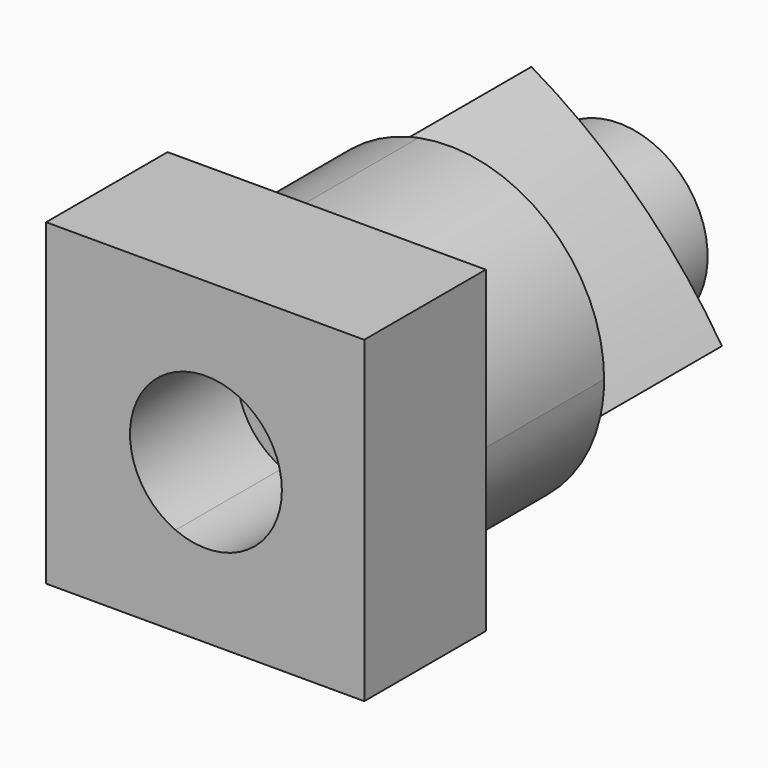
from build123d import *
from build123d import SkipClean  # not in build123d's __all__

# Parameters (mm, degrees)
F1_DEPTH = 6.35
F2_W     = 13.3050326258
F2_H     = 13.3050344884
F2_R     = 6.4893385046
F3_DEPTH = 6.35
F4_DEPTH = 25.4
F5_DEPTH = 7.112
F7_DEPTH = 6.35
F8_R     = 3.7056239581
F9_DEPTH = 2.54


# Not quite as in the source:
# - after a boolean that leaves OpenCascade's solid faulty, fix() repairs it


with BuildPart() as f1:
    # F0 (on Front) → F1 (new body)
    with BuildSketch(Plane.XZ):
        with BuildLine():
            ThreePointArc((-31.8034514785, 8.237525334), (-33.7084514785, 11.1474609002), (-31.8034514785, 14.0573964665))
            Line((-31.8034514785, 14.0573964665), (-31.8034514785, 17.5113130534))
            ThreePointArc((-31.8034514785, 17.5113130534), (-37.0227899831, 11.1474609002), (-31.8034514785, 4.7836087471))
            Line((-31.8034514785, 4.7836087471), (-31.8034514785, 8.237525334))
        make_face()
        with BuildLine():
            Line((-31.8034514785, 8.237525334), (-31.8034514785, 14.0573964665))
            ThreePointArc((-31.8034514785, 14.0573964665), (-33.7084514785, 11.1474609002), (-31.8034514785, 8.237525334))
        make_face()
        with BuildLine():
            ThreePointArc((-31.8034514785, 14.0573964665), (-28.7944323584, 13.8038564845), (-27.3584514785, 11.1474609002))
            ThreePointArc((-27.3584514785, 11.1474609002), (-28.7944323584, 8.491065316), (-31.8034514785, 8.237525334))
            Line((-31.8034514785, 8.237525334), (-31.8034514785, 4.7836087471))
            ThreePointArc((-31.8034514785, 4.7836087471), (-26.4182325094, 6.129843232), (-24.0441129739, 11.1474609002))
            ThreePointArc((-24.0441129739, 11.1474609002), (-26.4182325094, 16.1650785684), (-31.8034514785, 17.5113130534))
            Line((-31.8034514785, 17.5113130534), (-31.8034514785, 14.0573964665))
        make_face()
    extrude(amount=F1_DEPTH)

    # F2 (on face) → F3 (join)
    with BuildSketch(Plane.XZ.offset(6.35)):
        with Locations((-30.5656185374, 11.1557710916)):
            Rectangle(F2_W, F2_H)
        with Locations((-30.5334514785, 11.1474609002)):
            Circle(F2_R, mode=Mode.SUBTRACT)
        with Locations((-30.5334514785, 11.1474609002)):
            Circle(F2_R)
        with BuildLine():
            ThreePointArc((-31.8034514785, 14.0573964665), (-27.3584514785, 11.1474609002), (-31.8034514785, 8.237525334))
            Line((-31.8034514785, 8.237525334), (-31.8034514785, 14.0573964665))
        make_face(mode=Mode.SUBTRACT)
    extrude(amount=F3_DEPTH)

    # F0 (on Front) → F4 (cut)
    with BuildSketch(Plane.XZ):
        with BuildLine():
            Line((-31.8034514785, 8.237525334), (-31.8034514785, 14.0573964665))
            ThreePointArc((-31.8034514785, 14.0573964665), (-33.7084514785, 11.1474609002), (-31.8034514785, 8.237525334))
        make_face()
    extrude(amount=F4_DEPTH, mode=Mode.SUBTRACT)

    # F0 (on Front) → F5 (join)
    with BuildSketch(Plane.XZ):
        with BuildLine():
            Line((-31.8034514785, 8.237525334), (-31.8034514785, 14.0573964665))
            ThreePointArc((-31.8034514785, 14.0573964665), (-33.7084514785, 11.1474609002), (-31.8034514785, 8.237525334))
        make_face()
    extrude(amount=F5_DEPTH)

    # F6 (on face) → F7 (join)
    with BuildSketch(Plane(origin=(0, 0, 0), x_dir=(-1, 0, 0), z_dir=(0, 1, 0))):
        with BuildLine():
            ThreePointArc((32.1643167645, 17.4285271033), (27.7190855009, 14.0622502303), (24.1990881726, 9.7377248483))
            ThreePointArc((24.1990881726, 9.7377248483), (29.2426072016, 7.0222894593), (34.9343685496, 6.3784522862))
            ThreePointArc((34.9343685496, 6.3784522862), (34.7517106144, 12.2049013649), (32.1643167645, 17.4285271033))
        make_face()
        with BuildLine():
            Line((31.8034514785, 14.0573964665), (31.8034514785, 8.237525334))
            ThreePointArc((31.8034514785, 8.237525334), (27.3584514785, 11.1474609002), (31.8034514785, 14.0573964665))
        make_face(mode=Mode.SUBTRACT)
    with SkipClean():  # cleaning this boolean's faces spoils the solid; the shape is the same uncleaned
        extrude(amount=F7_DEPTH)

    # F8 (on face) → F9 (join)
    with BuildSketch(Plane(origin=(0, 6.35, 0), x_dir=(-1, 0, 0), z_dir=(0, 1, 0))):
        with Locations((30.5334514785, 11.1474609002)):
            Circle(F8_R)
        with BuildLine():
            ThreePointArc((31.8034514785, 8.237525334), (27.3584514785, 11.1474609002), (31.8034514785, 14.0573964665))
            Line((31.8034514785, 14.0573964665), (31.8034514785, 8.237525334))
        make_face(mode=Mode.SUBTRACT)
        with BuildLine():
            Line((31.8034514785, 8.237525334), (31.8034514785, 14.0573964665))
            ThreePointArc((31.8034514785, 14.0573964665), (27.3584514785, 11.1474609002), (31.8034514785, 8.237525334))
        make_face()
    extrude(amount=F9_DEPTH)

    add(f1.part.fix(), mode=Mode.REPLACE)


solid = f1.part
